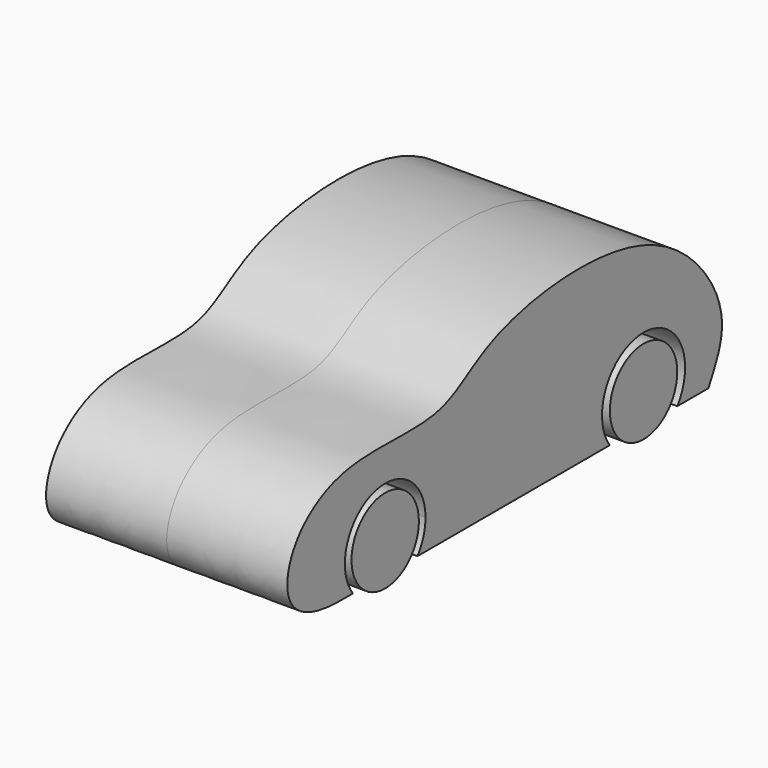
from build123d import *

# Parameters (mm, degrees)
F0_R     = 13.216614321
F1_DEPTH = 37.846


with BuildPart() as f1:
    # F0 (on Right) → F1 (new body, symmetric)
    with BuildSketch(Plane.YZ):
        with Locations((-50.6653307866, 13.5326530386)):
            Circle(F0_R)
    extrude(amount=F1_DEPTH, both=True)


with BuildPart() as f1b:
    # F0 (on Right) → F1, piece 2 (new body, symmetric)
    with BuildSketch(Plane.YZ):
        with Locations((50.6653307866, 13.5326530386)):
            Circle(F0_R)
    extrude(amount=F1_DEPTH, both=True)


with BuildPart() as f1c:
    # F0 (on Right) → F1, piece 3 (new body, symmetric)
    with BuildSketch(Plane.YZ):
        with BuildLine():
            ThreePointArc((-63.344253716, 4.0874228362), (-55.6407269298, 28.5397478089), (-34.8549715172, 13.5326530386))
            ThreePointArc((-34.8549715172, 13.5326530386), (-35.6582360163, 8.5572568954), (-37.9864078571, 4.0874228362))
            Line((-37.9864078571, 4.0874228362), (37.395499757, 4.0874228362))
            ThreePointArc((37.395499757, 4.0874228362), (45.707456761, 29.0478157602), (66.9533874273, 13.5326530386))
            ThreePointArc((66.9533874273, 13.5326530386), (66.1804935081, 8.574779013), (63.9351618162, 4.0874228362))
            Line((63.9351618162, 4.0874228362), (76.0923872439, 4.0874228362))
            add(Edge.make_bspline(
                [(-68.0214359061, 4.0874228362), (-87.9431305315, 4.0874228362), (-93.5747225099, 23.0474680653), (-68.9686816123, 44.1207693106), (-27.5033923902, 36.1284762743), (-10.3980912607, 56.2776935532), (56.5401787407, 63.1155509197), (86.5888672318, 23.4281355947), (79.4066745998, 10.1955566569), (76.0923872439, 4.0874228362)],
                knots=[0, 0, 0, 0, 0.1292301403, 0.2575864603, 0.4114148648, 0.5352528053, 0.730866763, 0.8908733985, 1, 1, 1, 1], degree=3))
            Line((-68.0214359061, 4.0874228362), (-63.344253716, 4.0874228362))
        make_face()
    extrude(amount=F1_DEPTH, both=True)


solid = Compound([f1.part, f1b.part, f1c.part])
